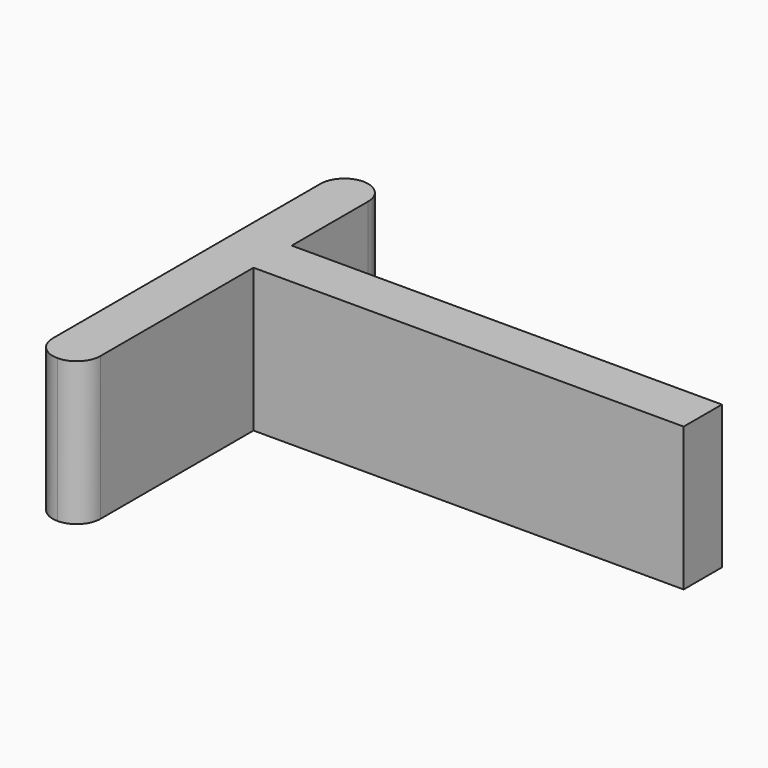
from build123d import *

# Parameters (mm, degrees)
F0_W     = 2
F0_H     = 5
F0_W_2   = 18
F0_H_2   = 2
F1_DEPTH = 6
F2_R     = 0.99999
F3_R     = 1
F4_R     = 0.99999


# Not quite as in the source:
# - a fillet or chamfer is up to 0.001 mm smaller than in the source, because OpenCascade refuses the exact size


with BuildPart() as f1:
    # F0 (on Top) → F1 (new body)
    with BuildSketch(Plane.XY):
        with Locations((1, 2.5)):
            Rectangle(F0_W, F0_H)
        with Locations((11, -1)):
            Rectangle(F0_W_2, F0_H_2)
        Polygon((2, 0), (0, 0), (0, -11), (2, -11), (2, -2), align=None)
    extrude(amount=F1_DEPTH)

    # F2 (radius 1 in the source; OpenCascade refuses exactly that, so slightly less here)
    f2_edges = [f1.edges().sort_by_distance(p)[0] for p in [
        (0, 5, 3),
        (2, 5, 3),
    ]]
    fillet(f2_edges, radius=F2_R)

    # F3
    f3_edges = [f1.edges().sort_by_distance(p)[0] for p in [
        (0, -11, 3),
    ]]
    fillet(f3_edges, radius=F3_R)

    # F4 (radius 1 in the source; OpenCascade refuses exactly that, so slightly less here)
    f4_edges = [f1.edges().sort_by_distance(p)[0] for p in [
        (2, -11, 3),
    ]]
    fillet(f4_edges, radius=F4_R)


solid = f1.part
